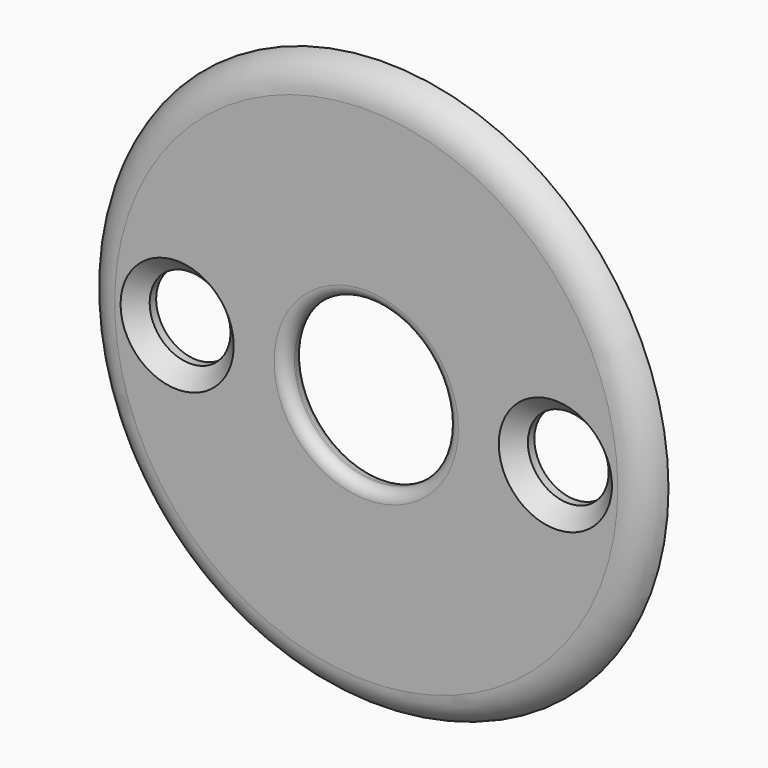
from build123d import *

# Parameters (mm, degrees)
F0_R           = 17.5
F0_R_2         = 5
F1_DEPTH       = 1.5
F2_D           = 5
F2_CSINK_D     = 7
F2_CSINK_ANGLE = 90
F4_R           = 0.7


# Not quite as in the source:
# - a fillet or chamfer that OpenCascade refuses, or shapes differently, is made with other operations: its cross-section is extruded or revolved along the edge and cut away or added


with BuildPart() as f1:
    # F0 (on Front) → F1 (new body)
    with BuildSketch(Plane.XZ):
        Circle(F0_R)
        Circle(F0_R_2, mode=Mode.SUBTRACT)
    extrude(amount=-F1_DEPTH)

    # F2 (through all)
    with Locations(Plane.XZ):
        with Locations((-11.7, 0), (11.7, 0)):
            CounterSinkHole(F2_D / 2, F2_CSINK_D / 2, counter_sink_angle=F2_CSINK_ANGLE)

    # F3: fillet of radius 2 on 1 edges, made by hand

    # F3_s1 → F3_t2 (revolve, cut)
    with BuildSketch(Plane.XY):
        with BuildLine():
            ThreePointArc((17.5, 1.5), (16.7882531983, 0.4188611699), (15.5635083269, 0))
            Line((15.5635083269, 0), (17.5, 0))
            Line((17.5, 0), (17.5, 1.5))
        make_face()
    revolve(axis=Axis((0, 0, 0), (0, -1, 0)), mode=Mode.SUBTRACT)

    # F4
    f4_edges = [f1.edges().sort_by_distance(p)[0] for p in [
        (-5, 0, 0),
        (-5, 1.5, 0),
    ]]
    fillet(f4_edges, radius=F4_R)


solid = f1.part
